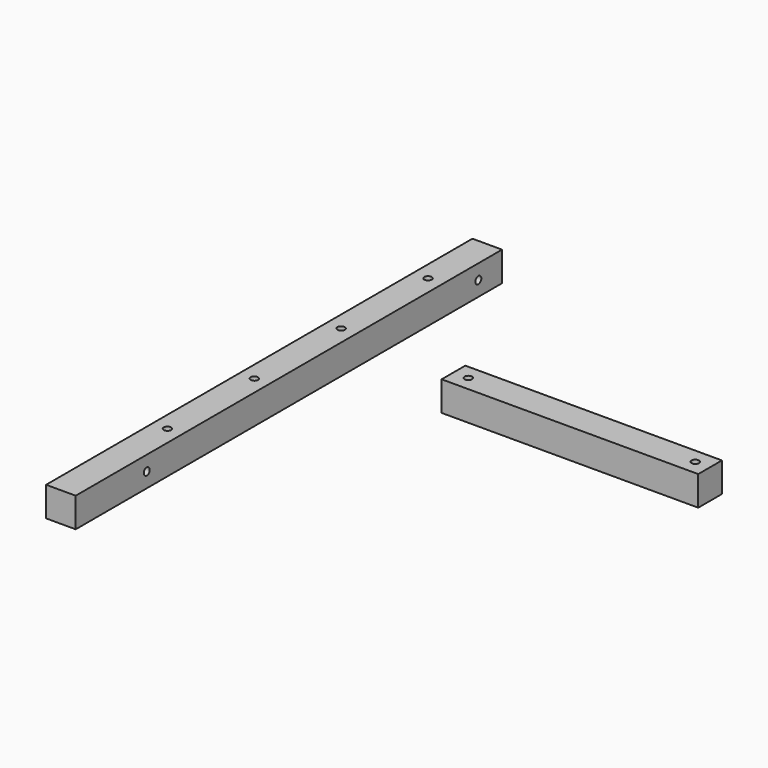
from build123d import *

# Parameters (mm, degrees)
F0_W      = 38.1
F0_H      = 685.8
F1_DEPTH  = 38.1
F4_D      = 9.525
F5_D      = 9.525
F6_D      = 9.525
F7_D      = 9.525
F8_D      = 9.525
F9_D      = 9.525
F10_W     = 330.2
F10_H     = 38.1
F11_DEPTH = 38.1
F12_D     = 9.525
F13_D     = 9.525


# Not quite as in the source:
# - a feature names something its author has since deleted; it is built from what else it names


with BuildPart() as f1:
    # F0 (on Top) → F1 (new body)
    with BuildSketch(Plane.XY):
        with Locations((1.3135822982, 35.9726289988)):
            Rectangle(F0_W, F0_H)
    extrude(amount=F1_DEPTH)

    # F4 (through all)
    with Locations(Plane(origin=(0, 0, 0), x_dir=(1, 0, 0), z_dir=(0, 0, -1))):
        with Locations((1.3135822982, 135.4773710012)):
            Hole(F4_D / 2)

    # F5 (through all)
    with Locations(Plane(origin=(0, 0, 0), x_dir=(1, 0, 0), z_dir=(0, 0, -1))):
        with Locations((1.3135822982, -4.2226289988)):
            Hole(F5_D / 2)

    # F6 (through all)
    with Locations(Plane(origin=(0, 0, 0), x_dir=(1, 0, 0), z_dir=(0, 0, -1))):
        with Locations((1.3135822982, -143.9226289988)):
            Hole(F6_D / 2)

    # F7 (through all)
    with Locations(Plane(origin=(0, 0, 0), x_dir=(1, 0, 0), z_dir=(0, 0, -1))):
        with Locations((1.3135822982, -283.6226289988)):
            Hole(F7_D / 2)

    # F8 (through all)
    with Locations(Plane.YZ.offset(20.3635822982)):
        with Locations((-192.6273710012, 19.05)):
            Hole(F8_D / 2)

    # F9 (through all)
    with Locations(Plane.YZ.offset(20.3635822982)):
        with Locations((340.7726289988, 19.05)):
            Hole(F9_D / 2)


with BuildPart() as f11:
    # F10 (on Top) → F11 (new body)
    with BuildSketch(Plane.XY):
        with Locations((314.3605970383, 139.6318280578)):
            Rectangle(F10_W, F10_H)
    extrude(amount=F11_DEPTH)

    # F12 (through all)
    with Locations(Plane(origin=(0, 0, 0), x_dir=(1, 0, 0), z_dir=(0, 0, -1))):
        with Locations((168.3105970383, -139.6318280578)):
            Hole(F12_D / 2)

    # F13 (through all)
    with Locations(Plane(origin=(0, 0, 0), x_dir=(1, 0, 0), z_dir=(0, 0, -1))):
        with Locations((460.4105970383, -139.6318280578)):
            Hole(F13_D / 2)


solid = Compound([f1.part, f11.part])
